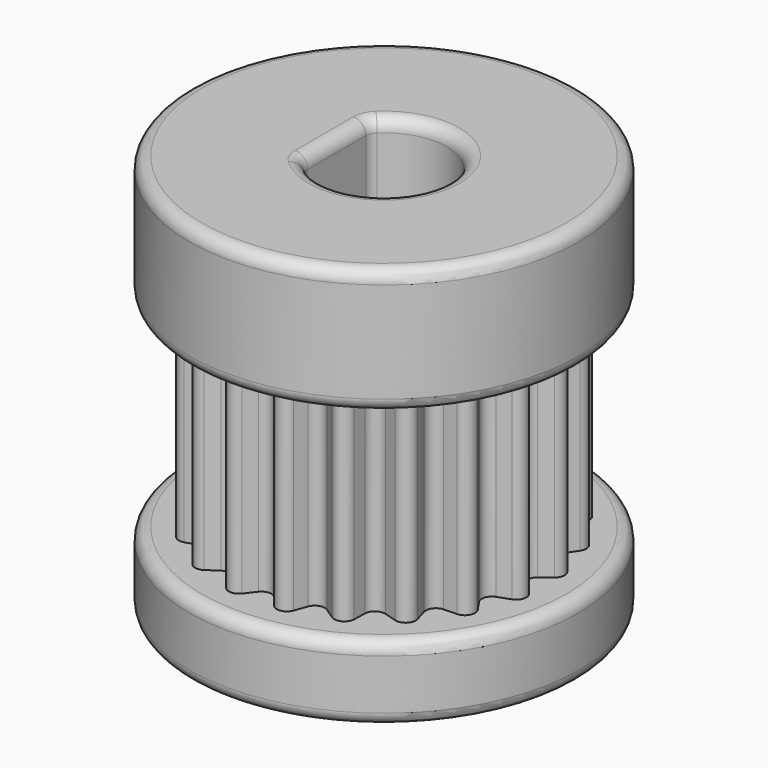
from build123d import *

# Parameters (mm, degrees)
F0_R     = 7.75
F1_DEPTH = 5
F2_DEPTH = 13
F3_START = -13
F3_DEPTH = 3
F4_R     = 0.5


with BuildPart() as f1:
    # F0 (on Top) → F1 (new body)
    with BuildSketch(Plane.XY):
        Circle(F0_R)
        with BuildLine():
            ThreePointArc((0.6382048465, 6.2700831172), (1.0168240228, 6.4199742139), (1.3305933613, 6.1604195498))
            Line((1.3305933613, 6.1604195498), (1.5086605411, 5.6659240772))
            ThreePointArc((1.5086605411, 5.6659240772), (1.7613968679, 5.4210221429), (2.1098145967, 5.4705972841))
            Line((2.1098145967, 5.4705972841), (2.5445311174, 5.7659872628))
            ThreePointArc((2.5445311174, 5.7659872628), (2.9509382483, 5.7915424072), (3.1691438202, 5.4477311947))
            Line((3.1691438202, 5.4477311947), (3.1856882672, 4.9224122685))
            ThreePointArc((3.1856882672, 4.9224122685), (3.3503759381, 4.6113968679), (3.6970604505, 4.5508786297))
            Line((3.6970604505, 4.5508786297), (4.2017809537, 4.6974764012))
            ThreePointArc((4.2017809537, 4.6974764012), (4.5961940777, 4.5961940777), (4.6974764012, 4.2017809537))
            Line((4.6974764012, 4.2017809537), (4.5508786297, 3.6970604505))
            ThreePointArc((4.5508786297, 3.6970604505), (4.6113968679, 3.3503759381), (4.9224122685, 3.1856882672))
            Line((4.9224122685, 3.1856882672), (5.4477311947, 3.1691438202))
            ThreePointArc((5.4477311947, 3.1691438202), (5.7915424072, 2.9509382483), (5.7659872628, 2.5445311174))
            Line((5.7659872628, 2.5445311174), (5.4705972841, 2.1098145967))
            ThreePointArc((5.4705972841, 2.1098145967), (5.4210221429, 1.7613968679), (5.6659240772, 1.5086605411))
            Line((5.6659240772, 1.5086605411), (6.1604195498, 1.3305933613))
            ThreePointArc((6.1604195498, 1.3305933613), (6.4199742139, 1.0168240228), (6.2700831172, 0.6382048465))
            Line((6.2700831172, 0.6382048465), (5.8548157604, 0.3160453902))
            ThreePointArc((5.8548157604, 0.3160453902), (5.7, 0), (5.8548157604, -0.3160453902))
            Line((5.8548157604, -0.3160453902), (6.2700831172, -0.6382048465))
            ThreePointArc((6.2700831172, -0.6382048465), (6.4199742139, -1.0168240228), (6.1604195498, -1.3305933613))
            Line((6.1604195498, -1.3305933613), (5.6659240772, -1.5086605411))
            ThreePointArc((5.6659240772, -1.5086605411), (5.4210221429, -1.7613968679), (5.4705972841, -2.1098145967))
            Line((5.4705972841, -2.1098145967), (5.7659872628, -2.5445311174))
            ThreePointArc((5.7659872628, -2.5445311174), (5.7915424072, -2.9509382483), (5.4477311947, -3.1691438202))
            Line((5.4477311947, -3.1691438202), (4.9224122685, -3.1856882672))
            ThreePointArc((4.9224122685, -3.1856882672), (4.6113968679, -3.3503759381), (4.5508786297, -3.6970604505))
            Line((4.5508786297, -3.6970604505), (4.6974764012, -4.2017809537))
            ThreePointArc((4.6974764012, -4.2017809537), (4.5961940777, -4.5961940777), (4.2017809537, -4.6974764012))
            Line((4.2017809537, -4.6974764012), (3.6970604505, -4.5508786297))
            ThreePointArc((3.6970604505, -4.5508786297), (3.3503759381, -4.6113968679), (3.1856882672, -4.9224122685))
            Line((3.1856882672, -4.9224122685), (3.1691438202, -5.4477311947))
            ThreePointArc((3.1691438202, -5.4477311947), (2.9509382483, -5.7915424072), (2.5445311174, -5.7659872628))
            Line((2.5445311174, -5.7659872628), (2.1098145967, -5.4705972841))
            ThreePointArc((2.1098145967, -5.4705972841), (1.7613968679, -5.4210221429), (1.5086605411, -5.6659240772))
            Line((1.5086605411, -5.6659240772), (1.3305933613, -6.1604195498))
            ThreePointArc((1.3305933613, -6.1604195498), (1.0168240228, -6.4199742139), (0.6382048465, -6.2700831172))
            Line((0.6382048465, -6.2700831172), (0.3160453902, -5.8548157604))
            ThreePointArc((0.3160453902, -5.8548157604), (0, -5.7), (-0.3160453902, -5.8548157604))
            Line((-0.3160453902, -5.8548157604), (-0.6382048465, -6.2700831172))
            ThreePointArc((-0.6382048465, -6.2700831172), (-1.0168240228, -6.4199742139), (-1.3305933613, -6.1604195498))
            Line((-1.3305933613, -6.1604195498), (-1.5086605411, -5.6659240772))
            ThreePointArc((-1.5086605411, -5.6659240772), (-1.7613968679, -5.4210221429), (-2.1098145967, -5.4705972841))
            Line((-2.1098145967, -5.4705972841), (-2.5445311174, -5.7659872628))
            ThreePointArc((-2.5445311174, -5.7659872628), (-2.9509382483, -5.7915424072), (-3.1691438202, -5.4477311947))
            Line((-3.1691438202, -5.4477311947), (-3.1856882672, -4.9224122685))
            ThreePointArc((-3.1856882672, -4.9224122685), (-3.3503759381, -4.6113968679), (-3.6970604505, -4.5508786297))
            Line((-3.6970604505, -4.5508786297), (-4.2017809537, -4.6974764012))
            ThreePointArc((-4.2017809537, -4.6974764012), (-4.5961940777, -4.5961940777), (-4.6974764012, -4.2017809537))
            Line((-4.6974764012, -4.2017809537), (-4.5508786297, -3.6970604505))
            ThreePointArc((-4.5508786297, -3.6970604505), (-4.6113968679, -3.3503759381), (-4.9224122685, -3.1856882672))
            Line((-4.9224122685, -3.1856882672), (-5.4477311947, -3.1691438202))
            ThreePointArc((-5.4477311947, -3.1691438202), (-5.7915424072, -2.9509382483), (-5.7659872628, -2.5445311174))
            Line((-5.7659872628, -2.5445311174), (-5.4705972841, -2.1098145967))
            ThreePointArc((-5.4705972841, -2.1098145967), (-5.4210221429, -1.7613968679), (-5.6659240772, -1.5086605411))
            Line((-5.6659240772, -1.5086605411), (-6.1604195498, -1.3305933613))
            ThreePointArc((-6.1604195498, -1.3305933613), (-6.4199742139, -1.0168240228), (-6.2700831172, -0.6382048465))
            Line((-6.2700831172, -0.6382048465), (-5.8548157604, -0.3160453902))
            ThreePointArc((-5.8548157604, -0.3160453902), (-5.7, 0), (-5.8548157604, 0.3160453902))
            Line((-5.8548157604, 0.3160453902), (-6.2700831172, 0.6382048465))
            ThreePointArc((-6.2700831172, 0.6382048465), (-6.4199742139, 1.0168240228), (-6.1604195498, 1.3305933613))
            Line((-6.1604195498, 1.3305933613), (-5.6659240772, 1.5086605411))
            ThreePointArc((-5.6659240772, 1.5086605411), (-5.4210221429, 1.7613968679), (-5.4705972841, 2.1098145967))
            Line((-5.4705972841, 2.1098145967), (-5.7659872628, 2.5445311174))
            ThreePointArc((-5.7659872628, 2.5445311174), (-5.7915424072, 2.9509382483), (-5.4477311947, 3.1691438202))
            Line((-5.4477311947, 3.1691438202), (-4.9224122685, 3.1856882672))
            ThreePointArc((-4.9224122685, 3.1856882672), (-4.6113968679, 3.3503759381), (-4.5508786297, 3.6970604505))
            Line((-4.5508786297, 3.6970604505), (-4.6974764012, 4.2017809537))
            ThreePointArc((-4.6974764012, 4.2017809537), (-4.5961940777, 4.5961940777), (-4.2017809537, 4.6974764012))
            Line((-4.2017809537, 4.6974764012), (-3.6970604505, 4.5508786297))
            ThreePointArc((-3.6970604505, 4.5508786297), (-3.3503759381, 4.6113968679), (-3.1856882672, 4.9224122685))
            Line((-3.1856882672, 4.9224122685), (-3.1691438202, 5.4477311947))
            ThreePointArc((-3.1691438202, 5.4477311947), (-2.9509382483, 5.7915424072), (-2.5445311174, 5.7659872628))
            Line((-2.5445311174, 5.7659872628), (-2.1098145967, 5.4705972841))
            ThreePointArc((-2.1098145967, 5.4705972841), (-1.7613968679, 5.4210221429), (-1.5086605411, 5.6659240772))
            Line((-1.5086605411, 5.6659240772), (-1.3305933613, 6.1604195498))
            ThreePointArc((-1.3305933613, 6.1604195498), (-1.0168240228, 6.4199742139), (-0.6382048465, 6.2700831172))
            Line((-0.6382048465, 6.2700831172), (-0.3160453902, 5.8548157604))
            ThreePointArc((-0.3160453902, 5.8548157604), (0, 5.7), (0.3160453902, 5.8548157604))
            Line((0.3160453902, 5.8548157604), (0.6382048465, 6.2700831172))
        make_face(mode=Mode.SUBTRACT)
        with BuildLine():
            Line((1.5086605411, 5.6659240772), (1.3305933613, 6.1604195498))
            ThreePointArc((1.3305933613, 6.1604195498), (1.0168240228, 6.4199742139), (0.6382048465, 6.2700831172))
            Line((0.6382048465, 6.2700831172), (0.3160453902, 5.8548157604))
            ThreePointArc((0.3160453902, 5.8548157604), (0, 5.7), (-0.3160453902, 5.8548157604))
            Line((-0.3160453902, 5.8548157604), (-0.6382048465, 6.2700831172))
            ThreePointArc((-0.6382048465, 6.2700831172), (-1.0168240228, 6.4199742139), (-1.3305933613, 6.1604195498))
            Line((-1.3305933613, 6.1604195498), (-1.5086605411, 5.6659240772))
            ThreePointArc((-1.5086605411, 5.6659240772), (-1.7613968679, 5.4210221429), (-2.1098145967, 5.4705972841))
            Line((-2.1098145967, 5.4705972841), (-2.5445311174, 5.7659872628))
            ThreePointArc((-2.5445311174, 5.7659872628), (-2.9509382483, 5.7915424072), (-3.1691438202, 5.4477311947))
            Line((-3.1691438202, 5.4477311947), (-3.1856882672, 4.9224122685))
            ThreePointArc((-3.1856882672, 4.9224122685), (-3.3503759381, 4.6113968679), (-3.6970604505, 4.5508786297))
            Line((-3.6970604505, 4.5508786297), (-4.2017809537, 4.6974764012))
            ThreePointArc((-4.2017809537, 4.6974764012), (-4.5961940777, 4.5961940777), (-4.6974764012, 4.2017809537))
            Line((-4.6974764012, 4.2017809537), (-4.5508786297, 3.6970604505))
            ThreePointArc((-4.5508786297, 3.6970604505), (-4.6113968679, 3.3503759381), (-4.9224122685, 3.1856882672))
            Line((-4.9224122685, 3.1856882672), (-5.4477311947, 3.1691438202))
            ThreePointArc((-5.4477311947, 3.1691438202), (-5.7915424072, 2.9509382483), (-5.7659872628, 2.5445311174))
            Line((-5.7659872628, 2.5445311174), (-5.4705972841, 2.1098145967))
            ThreePointArc((-5.4705972841, 2.1098145967), (-5.4210221429, 1.7613968679), (-5.6659240772, 1.5086605411))
            Line((-5.6659240772, 1.5086605411), (-6.1604195498, 1.3305933613))
            ThreePointArc((-6.1604195498, 1.3305933613), (-6.4199742139, 1.0168240228), (-6.2700831172, 0.6382048465))
            Line((-6.2700831172, 0.6382048465), (-5.8548157604, 0.3160453902))
            ThreePointArc((-5.8548157604, 0.3160453902), (-5.7, 0), (-5.8548157604, -0.3160453902))
            Line((-5.8548157604, -0.3160453902), (-6.2700831172, -0.6382048465))
            ThreePointArc((-6.2700831172, -0.6382048465), (-6.4199742139, -1.0168240228), (-6.1604195498, -1.3305933613))
            Line((-6.1604195498, -1.3305933613), (-5.6659240772, -1.5086605411))
            ThreePointArc((-5.6659240772, -1.5086605411), (-5.4210221429, -1.7613968679), (-5.4705972841, -2.1098145967))
            Line((-5.4705972841, -2.1098145967), (-5.7659872628, -2.5445311174))
            ThreePointArc((-5.7659872628, -2.5445311174), (-5.7915424072, -2.9509382483), (-5.4477311947, -3.1691438202))
            Line((-5.4477311947, -3.1691438202), (-4.9224122685, -3.1856882672))
            ThreePointArc((-4.9224122685, -3.1856882672), (-4.6113968679, -3.3503759381), (-4.5508786297, -3.6970604505))
            Line((-4.5508786297, -3.6970604505), (-4.6974764012, -4.2017809537))
            ThreePointArc((-4.6974764012, -4.2017809537), (-4.5961940777, -4.5961940777), (-4.2017809537, -4.6974764012))
            Line((-4.2017809537, -4.6974764012), (-3.6970604505, -4.5508786297))
            ThreePointArc((-3.6970604505, -4.5508786297), (-3.3503759381, -4.6113968679), (-3.1856882672, -4.9224122685))
            Line((-3.1856882672, -4.9224122685), (-3.1691438202, -5.4477311947))
            ThreePointArc((-3.1691438202, -5.4477311947), (-2.9509382483, -5.7915424072), (-2.5445311174, -5.7659872628))
            Line((-2.5445311174, -5.7659872628), (-2.1098145967, -5.4705972841))
            ThreePointArc((-2.1098145967, -5.4705972841), (-1.7613968679, -5.4210221429), (-1.5086605411, -5.6659240772))
            Line((-1.5086605411, -5.6659240772), (-1.3305933613, -6.1604195498))
            ThreePointArc((-1.3305933613, -6.1604195498), (-1.0168240228, -6.4199742139), (-0.6382048465, -6.2700831172))
            Line((-0.6382048465, -6.2700831172), (-0.3160453902, -5.8548157604))
            ThreePointArc((-0.3160453902, -5.8548157604), (0, -5.7), (0.3160453902, -5.8548157604))
            Line((0.3160453902, -5.8548157604), (0.6382048465, -6.2700831172))
            ThreePointArc((0.6382048465, -6.2700831172), (1.0168240228, -6.4199742139), (1.3305933613, -6.1604195498))
            Line((1.3305933613, -6.1604195498), (1.5086605411, -5.6659240772))
            ThreePointArc((1.5086605411, -5.6659240772), (1.7613968679, -5.4210221429), (2.1098145967, -5.4705972841))
            Line((2.1098145967, -5.4705972841), (2.5445311174, -5.7659872628))
            ThreePointArc((2.5445311174, -5.7659872628), (2.9509382483, -5.7915424072), (3.1691438202, -5.4477311947))
            Line((3.1691438202, -5.4477311947), (3.1856882672, -4.9224122685))
            ThreePointArc((3.1856882672, -4.9224122685), (3.3503759381, -4.6113968679), (3.6970604505, -4.5508786297))
            Line((3.6970604505, -4.5508786297), (4.2017809537, -4.6974764012))
            ThreePointArc((4.2017809537, -4.6974764012), (4.5961940777, -4.5961940777), (4.6974764012, -4.2017809537))
            Line((4.6974764012, -4.2017809537), (4.5508786297, -3.6970604505))
            ThreePointArc((4.5508786297, -3.6970604505), (4.6113968679, -3.3503759381), (4.9224122685, -3.1856882672))
            Line((4.9224122685, -3.1856882672), (5.4477311947, -3.1691438202))
            ThreePointArc((5.4477311947, -3.1691438202), (5.7915424072, -2.9509382483), (5.7659872628, -2.5445311174))
            Line((5.7659872628, -2.5445311174), (5.4705972841, -2.1098145967))
            ThreePointArc((5.4705972841, -2.1098145967), (5.4210221429, -1.7613968679), (5.6659240772, -1.5086605411))
            Line((5.6659240772, -1.5086605411), (6.1604195498, -1.3305933613))
            ThreePointArc((6.1604195498, -1.3305933613), (6.4199742139, -1.0168240228), (6.2700831172, -0.6382048465))
            Line((6.2700831172, -0.6382048465), (5.8548157604, -0.3160453902))
            ThreePointArc((5.8548157604, -0.3160453902), (5.7, 0), (5.8548157604, 0.3160453902))
            Line((5.8548157604, 0.3160453902), (6.2700831172, 0.6382048465))
            ThreePointArc((6.2700831172, 0.6382048465), (6.4199742139, 1.0168240228), (6.1604195498, 1.3305933613))
            Line((6.1604195498, 1.3305933613), (5.6659240772, 1.5086605411))
            ThreePointArc((5.6659240772, 1.5086605411), (5.4210221429, 1.7613968679), (5.4705972841, 2.1098145967))
            Line((5.4705972841, 2.1098145967), (5.7659872628, 2.5445311174))
            ThreePointArc((5.7659872628, 2.5445311174), (5.7915424072, 2.9509382483), (5.4477311947, 3.1691438202))
            Line((5.4477311947, 3.1691438202), (4.9224122685, 3.1856882672))
            ThreePointArc((4.9224122685, 3.1856882672), (4.6113968679, 3.3503759381), (4.5508786297, 3.6970604505))
            Line((4.5508786297, 3.6970604505), (4.6974764012, 4.2017809537))
            ThreePointArc((4.6974764012, 4.2017809537), (4.5961940777, 4.5961940777), (4.2017809537, 4.6974764012))
            Line((4.2017809537, 4.6974764012), (3.6970604505, 4.5508786297))
            ThreePointArc((3.6970604505, 4.5508786297), (3.3503759381, 4.6113968679), (3.1856882672, 4.9224122685))
            Line((3.1856882672, 4.9224122685), (3.1691438202, 5.4477311947))
            ThreePointArc((3.1691438202, 5.4477311947), (2.9509382483, 5.7915424072), (2.5445311174, 5.7659872628))
            Line((2.5445311174, 5.7659872628), (2.1098145967, 5.4705972841))
            ThreePointArc((2.1098145967, 5.4705972841), (1.7613968679, 5.4210221429), (1.5086605411, 5.6659240772))
        make_face()
        with BuildLine():
            ThreePointArc((-1.8781639971, 1.65), (2.5, 0), (-1.8781639971, -1.65))
            Line((-1.8781639971, -1.65), (-1.8781639971, 1.65))
        make_face(mode=Mode.SUBTRACT)
    extrude(amount=-F1_DEPTH)

    # F0 (on Top) → F2 (join)
    with BuildSketch(Plane.XY):
        with BuildLine():
            Line((1.5086605411, 5.6659240772), (1.3305933613, 6.1604195498))
            ThreePointArc((1.3305933613, 6.1604195498), (1.0168240228, 6.4199742139), (0.6382048465, 6.2700831172))
            Line((0.6382048465, 6.2700831172), (0.3160453902, 5.8548157604))
            ThreePointArc((0.3160453902, 5.8548157604), (0, 5.7), (-0.3160453902, 5.8548157604))
            Line((-0.3160453902, 5.8548157604), (-0.6382048465, 6.2700831172))
            ThreePointArc((-0.6382048465, 6.2700831172), (-1.0168240228, 6.4199742139), (-1.3305933613, 6.1604195498))
            Line((-1.3305933613, 6.1604195498), (-1.5086605411, 5.6659240772))
            ThreePointArc((-1.5086605411, 5.6659240772), (-1.7613968679, 5.4210221429), (-2.1098145967, 5.4705972841))
            Line((-2.1098145967, 5.4705972841), (-2.5445311174, 5.7659872628))
            ThreePointArc((-2.5445311174, 5.7659872628), (-2.9509382483, 5.7915424072), (-3.1691438202, 5.4477311947))
            Line((-3.1691438202, 5.4477311947), (-3.1856882672, 4.9224122685))
            ThreePointArc((-3.1856882672, 4.9224122685), (-3.3503759381, 4.6113968679), (-3.6970604505, 4.5508786297))
            Line((-3.6970604505, 4.5508786297), (-4.2017809537, 4.6974764012))
            ThreePointArc((-4.2017809537, 4.6974764012), (-4.5961940777, 4.5961940777), (-4.6974764012, 4.2017809537))
            Line((-4.6974764012, 4.2017809537), (-4.5508786297, 3.6970604505))
            ThreePointArc((-4.5508786297, 3.6970604505), (-4.6113968679, 3.3503759381), (-4.9224122685, 3.1856882672))
            Line((-4.9224122685, 3.1856882672), (-5.4477311947, 3.1691438202))
            ThreePointArc((-5.4477311947, 3.1691438202), (-5.7915424072, 2.9509382483), (-5.7659872628, 2.5445311174))
            Line((-5.7659872628, 2.5445311174), (-5.4705972841, 2.1098145967))
            ThreePointArc((-5.4705972841, 2.1098145967), (-5.4210221429, 1.7613968679), (-5.6659240772, 1.5086605411))
            Line((-5.6659240772, 1.5086605411), (-6.1604195498, 1.3305933613))
            ThreePointArc((-6.1604195498, 1.3305933613), (-6.4199742139, 1.0168240228), (-6.2700831172, 0.6382048465))
            Line((-6.2700831172, 0.6382048465), (-5.8548157604, 0.3160453902))
            ThreePointArc((-5.8548157604, 0.3160453902), (-5.7, 0), (-5.8548157604, -0.3160453902))
            Line((-5.8548157604, -0.3160453902), (-6.2700831172, -0.6382048465))
            ThreePointArc((-6.2700831172, -0.6382048465), (-6.4199742139, -1.0168240228), (-6.1604195498, -1.3305933613))
            Line((-6.1604195498, -1.3305933613), (-5.6659240772, -1.5086605411))
            ThreePointArc((-5.6659240772, -1.5086605411), (-5.4210221429, -1.7613968679), (-5.4705972841, -2.1098145967))
            Line((-5.4705972841, -2.1098145967), (-5.7659872628, -2.5445311174))
            ThreePointArc((-5.7659872628, -2.5445311174), (-5.7915424072, -2.9509382483), (-5.4477311947, -3.1691438202))
            Line((-5.4477311947, -3.1691438202), (-4.9224122685, -3.1856882672))
            ThreePointArc((-4.9224122685, -3.1856882672), (-4.6113968679, -3.3503759381), (-4.5508786297, -3.6970604505))
            Line((-4.5508786297, -3.6970604505), (-4.6974764012, -4.2017809537))
            ThreePointArc((-4.6974764012, -4.2017809537), (-4.5961940777, -4.5961940777), (-4.2017809537, -4.6974764012))
            Line((-4.2017809537, -4.6974764012), (-3.6970604505, -4.5508786297))
            ThreePointArc((-3.6970604505, -4.5508786297), (-3.3503759381, -4.6113968679), (-3.1856882672, -4.9224122685))
            Line((-3.1856882672, -4.9224122685), (-3.1691438202, -5.4477311947))
            ThreePointArc((-3.1691438202, -5.4477311947), (-2.9509382483, -5.7915424072), (-2.5445311174, -5.7659872628))
            Line((-2.5445311174, -5.7659872628), (-2.1098145967, -5.4705972841))
            ThreePointArc((-2.1098145967, -5.4705972841), (-1.7613968679, -5.4210221429), (-1.5086605411, -5.6659240772))
            Line((-1.5086605411, -5.6659240772), (-1.3305933613, -6.1604195498))
            ThreePointArc((-1.3305933613, -6.1604195498), (-1.0168240228, -6.4199742139), (-0.6382048465, -6.2700831172))
            Line((-0.6382048465, -6.2700831172), (-0.3160453902, -5.8548157604))
            ThreePointArc((-0.3160453902, -5.8548157604), (0, -5.7), (0.3160453902, -5.8548157604))
            Line((0.3160453902, -5.8548157604), (0.6382048465, -6.2700831172))
            ThreePointArc((0.6382048465, -6.2700831172), (1.0168240228, -6.4199742139), (1.3305933613, -6.1604195498))
            Line((1.3305933613, -6.1604195498), (1.5086605411, -5.6659240772))
            ThreePointArc((1.5086605411, -5.6659240772), (1.7613968679, -5.4210221429), (2.1098145967, -5.4705972841))
            Line((2.1098145967, -5.4705972841), (2.5445311174, -5.7659872628))
            ThreePointArc((2.5445311174, -5.7659872628), (2.9509382483, -5.7915424072), (3.1691438202, -5.4477311947))
            Line((3.1691438202, -5.4477311947), (3.1856882672, -4.9224122685))
            ThreePointArc((3.1856882672, -4.9224122685), (3.3503759381, -4.6113968679), (3.6970604505, -4.5508786297))
            Line((3.6970604505, -4.5508786297), (4.2017809537, -4.6974764012))
            ThreePointArc((4.2017809537, -4.6974764012), (4.5961940777, -4.5961940777), (4.6974764012, -4.2017809537))
            Line((4.6974764012, -4.2017809537), (4.5508786297, -3.6970604505))
            ThreePointArc((4.5508786297, -3.6970604505), (4.6113968679, -3.3503759381), (4.9224122685, -3.1856882672))
            Line((4.9224122685, -3.1856882672), (5.4477311947, -3.1691438202))
            ThreePointArc((5.4477311947, -3.1691438202), (5.7915424072, -2.9509382483), (5.7659872628, -2.5445311174))
            Line((5.7659872628, -2.5445311174), (5.4705972841, -2.1098145967))
            ThreePointArc((5.4705972841, -2.1098145967), (5.4210221429, -1.7613968679), (5.6659240772, -1.5086605411))
            Line((5.6659240772, -1.5086605411), (6.1604195498, -1.3305933613))
            ThreePointArc((6.1604195498, -1.3305933613), (6.4199742139, -1.0168240228), (6.2700831172, -0.6382048465))
            Line((6.2700831172, -0.6382048465), (5.8548157604, -0.3160453902))
            ThreePointArc((5.8548157604, -0.3160453902), (5.7, 0), (5.8548157604, 0.3160453902))
            Line((5.8548157604, 0.3160453902), (6.2700831172, 0.6382048465))
            ThreePointArc((6.2700831172, 0.6382048465), (6.4199742139, 1.0168240228), (6.1604195498, 1.3305933613))
            Line((6.1604195498, 1.3305933613), (5.6659240772, 1.5086605411))
            ThreePointArc((5.6659240772, 1.5086605411), (5.4210221429, 1.7613968679), (5.4705972841, 2.1098145967))
            Line((5.4705972841, 2.1098145967), (5.7659872628, 2.5445311174))
            ThreePointArc((5.7659872628, 2.5445311174), (5.7915424072, 2.9509382483), (5.4477311947, 3.1691438202))
            Line((5.4477311947, 3.1691438202), (4.9224122685, 3.1856882672))
            ThreePointArc((4.9224122685, 3.1856882672), (4.6113968679, 3.3503759381), (4.5508786297, 3.6970604505))
            Line((4.5508786297, 3.6970604505), (4.6974764012, 4.2017809537))
            ThreePointArc((4.6974764012, 4.2017809537), (4.5961940777, 4.5961940777), (4.2017809537, 4.6974764012))
            Line((4.2017809537, 4.6974764012), (3.6970604505, 4.5508786297))
            ThreePointArc((3.6970604505, 4.5508786297), (3.3503759381, 4.6113968679), (3.1856882672, 4.9224122685))
            Line((3.1856882672, 4.9224122685), (3.1691438202, 5.4477311947))
            ThreePointArc((3.1691438202, 5.4477311947), (2.9509382483, 5.7915424072), (2.5445311174, 5.7659872628))
            Line((2.5445311174, 5.7659872628), (2.1098145967, 5.4705972841))
            ThreePointArc((2.1098145967, 5.4705972841), (1.7613968679, 5.4210221429), (1.5086605411, 5.6659240772))
        make_face()
        with BuildLine():
            ThreePointArc((-1.8781639971, 1.65), (2.5, 0), (-1.8781639971, -1.65))
            Line((-1.8781639971, -1.65), (-1.8781639971, 1.65))
        make_face(mode=Mode.SUBTRACT)
    extrude(amount=-F2_DEPTH)

    # F0 (on Top) → F3 (join)
    with BuildSketch(Plane.XY.offset(F3_START)):
        Circle(F0_R)
        with BuildLine():
            ThreePointArc((0.6382048465, 6.2700831172), (1.0168240228, 6.4199742139), (1.3305933613, 6.1604195498))
            Line((1.3305933613, 6.1604195498), (1.5086605411, 5.6659240772))
            ThreePointArc((1.5086605411, 5.6659240772), (1.7613968679, 5.4210221429), (2.1098145967, 5.4705972841))
            Line((2.1098145967, 5.4705972841), (2.5445311174, 5.7659872628))
            ThreePointArc((2.5445311174, 5.7659872628), (2.9509382483, 5.7915424072), (3.1691438202, 5.4477311947))
            Line((3.1691438202, 5.4477311947), (3.1856882672, 4.9224122685))
            ThreePointArc((3.1856882672, 4.9224122685), (3.3503759381, 4.6113968679), (3.6970604505, 4.5508786297))
            Line((3.6970604505, 4.5508786297), (4.2017809537, 4.6974764012))
            ThreePointArc((4.2017809537, 4.6974764012), (4.5961940777, 4.5961940777), (4.6974764012, 4.2017809537))
            Line((4.6974764012, 4.2017809537), (4.5508786297, 3.6970604505))
            ThreePointArc((4.5508786297, 3.6970604505), (4.6113968679, 3.3503759381), (4.9224122685, 3.1856882672))
            Line((4.9224122685, 3.1856882672), (5.4477311947, 3.1691438202))
            ThreePointArc((5.4477311947, 3.1691438202), (5.7915424072, 2.9509382483), (5.7659872628, 2.5445311174))
            Line((5.7659872628, 2.5445311174), (5.4705972841, 2.1098145967))
            ThreePointArc((5.4705972841, 2.1098145967), (5.4210221429, 1.7613968679), (5.6659240772, 1.5086605411))
            Line((5.6659240772, 1.5086605411), (6.1604195498, 1.3305933613))
            ThreePointArc((6.1604195498, 1.3305933613), (6.4199742139, 1.0168240228), (6.2700831172, 0.6382048465))
            Line((6.2700831172, 0.6382048465), (5.8548157604, 0.3160453902))
            ThreePointArc((5.8548157604, 0.3160453902), (5.7, 0), (5.8548157604, -0.3160453902))
            Line((5.8548157604, -0.3160453902), (6.2700831172, -0.6382048465))
            ThreePointArc((6.2700831172, -0.6382048465), (6.4199742139, -1.0168240228), (6.1604195498, -1.3305933613))
            Line((6.1604195498, -1.3305933613), (5.6659240772, -1.5086605411))
            ThreePointArc((5.6659240772, -1.5086605411), (5.4210221429, -1.7613968679), (5.4705972841, -2.1098145967))
            Line((5.4705972841, -2.1098145967), (5.7659872628, -2.5445311174))
            ThreePointArc((5.7659872628, -2.5445311174), (5.7915424072, -2.9509382483), (5.4477311947, -3.1691438202))
            Line((5.4477311947, -3.1691438202), (4.9224122685, -3.1856882672))
            ThreePointArc((4.9224122685, -3.1856882672), (4.6113968679, -3.3503759381), (4.5508786297, -3.6970604505))
            Line((4.5508786297, -3.6970604505), (4.6974764012, -4.2017809537))
            ThreePointArc((4.6974764012, -4.2017809537), (4.5961940777, -4.5961940777), (4.2017809537, -4.6974764012))
            Line((4.2017809537, -4.6974764012), (3.6970604505, -4.5508786297))
            ThreePointArc((3.6970604505, -4.5508786297), (3.3503759381, -4.6113968679), (3.1856882672, -4.9224122685))
            Line((3.1856882672, -4.9224122685), (3.1691438202, -5.4477311947))
            ThreePointArc((3.1691438202, -5.4477311947), (2.9509382483, -5.7915424072), (2.5445311174, -5.7659872628))
            Line((2.5445311174, -5.7659872628), (2.1098145967, -5.4705972841))
            ThreePointArc((2.1098145967, -5.4705972841), (1.7613968679, -5.4210221429), (1.5086605411, -5.6659240772))
            Line((1.5086605411, -5.6659240772), (1.3305933613, -6.1604195498))
            ThreePointArc((1.3305933613, -6.1604195498), (1.0168240228, -6.4199742139), (0.6382048465, -6.2700831172))
            Line((0.6382048465, -6.2700831172), (0.3160453902, -5.8548157604))
            ThreePointArc((0.3160453902, -5.8548157604), (0, -5.7), (-0.3160453902, -5.8548157604))
            Line((-0.3160453902, -5.8548157604), (-0.6382048465, -6.2700831172))
            ThreePointArc((-0.6382048465, -6.2700831172), (-1.0168240228, -6.4199742139), (-1.3305933613, -6.1604195498))
            Line((-1.3305933613, -6.1604195498), (-1.5086605411, -5.6659240772))
            ThreePointArc((-1.5086605411, -5.6659240772), (-1.7613968679, -5.4210221429), (-2.1098145967, -5.4705972841))
            Line((-2.1098145967, -5.4705972841), (-2.5445311174, -5.7659872628))
            ThreePointArc((-2.5445311174, -5.7659872628), (-2.9509382483, -5.7915424072), (-3.1691438202, -5.4477311947))
            Line((-3.1691438202, -5.4477311947), (-3.1856882672, -4.9224122685))
            ThreePointArc((-3.1856882672, -4.9224122685), (-3.3503759381, -4.6113968679), (-3.6970604505, -4.5508786297))
            Line((-3.6970604505, -4.5508786297), (-4.2017809537, -4.6974764012))
            ThreePointArc((-4.2017809537, -4.6974764012), (-4.5961940777, -4.5961940777), (-4.6974764012, -4.2017809537))
            Line((-4.6974764012, -4.2017809537), (-4.5508786297, -3.6970604505))
            ThreePointArc((-4.5508786297, -3.6970604505), (-4.6113968679, -3.3503759381), (-4.9224122685, -3.1856882672))
            Line((-4.9224122685, -3.1856882672), (-5.4477311947, -3.1691438202))
            ThreePointArc((-5.4477311947, -3.1691438202), (-5.7915424072, -2.9509382483), (-5.7659872628, -2.5445311174))
            Line((-5.7659872628, -2.5445311174), (-5.4705972841, -2.1098145967))
            ThreePointArc((-5.4705972841, -2.1098145967), (-5.4210221429, -1.7613968679), (-5.6659240772, -1.5086605411))
            Line((-5.6659240772, -1.5086605411), (-6.1604195498, -1.3305933613))
            ThreePointArc((-6.1604195498, -1.3305933613), (-6.4199742139, -1.0168240228), (-6.2700831172, -0.6382048465))
            Line((-6.2700831172, -0.6382048465), (-5.8548157604, -0.3160453902))
            ThreePointArc((-5.8548157604, -0.3160453902), (-5.7, 0), (-5.8548157604, 0.3160453902))
            Line((-5.8548157604, 0.3160453902), (-6.2700831172, 0.6382048465))
            ThreePointArc((-6.2700831172, 0.6382048465), (-6.4199742139, 1.0168240228), (-6.1604195498, 1.3305933613))
            Line((-6.1604195498, 1.3305933613), (-5.6659240772, 1.5086605411))
            ThreePointArc((-5.6659240772, 1.5086605411), (-5.4210221429, 1.7613968679), (-5.4705972841, 2.1098145967))
            Line((-5.4705972841, 2.1098145967), (-5.7659872628, 2.5445311174))
            ThreePointArc((-5.7659872628, 2.5445311174), (-5.7915424072, 2.9509382483), (-5.4477311947, 3.1691438202))
            Line((-5.4477311947, 3.1691438202), (-4.9224122685, 3.1856882672))
            ThreePointArc((-4.9224122685, 3.1856882672), (-4.6113968679, 3.3503759381), (-4.5508786297, 3.6970604505))
            Line((-4.5508786297, 3.6970604505), (-4.6974764012, 4.2017809537))
            ThreePointArc((-4.6974764012, 4.2017809537), (-4.5961940777, 4.5961940777), (-4.2017809537, 4.6974764012))
            Line((-4.2017809537, 4.6974764012), (-3.6970604505, 4.5508786297))
            ThreePointArc((-3.6970604505, 4.5508786297), (-3.3503759381, 4.6113968679), (-3.1856882672, 4.9224122685))
            Line((-3.1856882672, 4.9224122685), (-3.1691438202, 5.4477311947))
            ThreePointArc((-3.1691438202, 5.4477311947), (-2.9509382483, 5.7915424072), (-2.5445311174, 5.7659872628))
            Line((-2.5445311174, 5.7659872628), (-2.1098145967, 5.4705972841))
            ThreePointArc((-2.1098145967, 5.4705972841), (-1.7613968679, 5.4210221429), (-1.5086605411, 5.6659240772))
            Line((-1.5086605411, 5.6659240772), (-1.3305933613, 6.1604195498))
            ThreePointArc((-1.3305933613, 6.1604195498), (-1.0168240228, 6.4199742139), (-0.6382048465, 6.2700831172))
            Line((-0.6382048465, 6.2700831172), (-0.3160453902, 5.8548157604))
            ThreePointArc((-0.3160453902, 5.8548157604), (0, 5.7), (0.3160453902, 5.8548157604))
            Line((0.3160453902, 5.8548157604), (0.6382048465, 6.2700831172))
        make_face(mode=Mode.SUBTRACT)
        with BuildLine():
            Line((1.5086605411, 5.6659240772), (1.3305933613, 6.1604195498))
            ThreePointArc((1.3305933613, 6.1604195498), (1.0168240228, 6.4199742139), (0.6382048465, 6.2700831172))
            Line((0.6382048465, 6.2700831172), (0.3160453902, 5.8548157604))
            ThreePointArc((0.3160453902, 5.8548157604), (0, 5.7), (-0.3160453902, 5.8548157604))
            Line((-0.3160453902, 5.8548157604), (-0.6382048465, 6.2700831172))
            ThreePointArc((-0.6382048465, 6.2700831172), (-1.0168240228, 6.4199742139), (-1.3305933613, 6.1604195498))
            Line((-1.3305933613, 6.1604195498), (-1.5086605411, 5.6659240772))
            ThreePointArc((-1.5086605411, 5.6659240772), (-1.7613968679, 5.4210221429), (-2.1098145967, 5.4705972841))
            Line((-2.1098145967, 5.4705972841), (-2.5445311174, 5.7659872628))
            ThreePointArc((-2.5445311174, 5.7659872628), (-2.9509382483, 5.7915424072), (-3.1691438202, 5.4477311947))
            Line((-3.1691438202, 5.4477311947), (-3.1856882672, 4.9224122685))
            ThreePointArc((-3.1856882672, 4.9224122685), (-3.3503759381, 4.6113968679), (-3.6970604505, 4.5508786297))
            Line((-3.6970604505, 4.5508786297), (-4.2017809537, 4.6974764012))
            ThreePointArc((-4.2017809537, 4.6974764012), (-4.5961940777, 4.5961940777), (-4.6974764012, 4.2017809537))
            Line((-4.6974764012, 4.2017809537), (-4.5508786297, 3.6970604505))
            ThreePointArc((-4.5508786297, 3.6970604505), (-4.6113968679, 3.3503759381), (-4.9224122685, 3.1856882672))
            Line((-4.9224122685, 3.1856882672), (-5.4477311947, 3.1691438202))
            ThreePointArc((-5.4477311947, 3.1691438202), (-5.7915424072, 2.9509382483), (-5.7659872628, 2.5445311174))
            Line((-5.7659872628, 2.5445311174), (-5.4705972841, 2.1098145967))
            ThreePointArc((-5.4705972841, 2.1098145967), (-5.4210221429, 1.7613968679), (-5.6659240772, 1.5086605411))
            Line((-5.6659240772, 1.5086605411), (-6.1604195498, 1.3305933613))
            ThreePointArc((-6.1604195498, 1.3305933613), (-6.4199742139, 1.0168240228), (-6.2700831172, 0.6382048465))
            Line((-6.2700831172, 0.6382048465), (-5.8548157604, 0.3160453902))
            ThreePointArc((-5.8548157604, 0.3160453902), (-5.7, 0), (-5.8548157604, -0.3160453902))
            Line((-5.8548157604, -0.3160453902), (-6.2700831172, -0.6382048465))
            ThreePointArc((-6.2700831172, -0.6382048465), (-6.4199742139, -1.0168240228), (-6.1604195498, -1.3305933613))
            Line((-6.1604195498, -1.3305933613), (-5.6659240772, -1.5086605411))
            ThreePointArc((-5.6659240772, -1.5086605411), (-5.4210221429, -1.7613968679), (-5.4705972841, -2.1098145967))
            Line((-5.4705972841, -2.1098145967), (-5.7659872628, -2.5445311174))
            ThreePointArc((-5.7659872628, -2.5445311174), (-5.7915424072, -2.9509382483), (-5.4477311947, -3.1691438202))
            Line((-5.4477311947, -3.1691438202), (-4.9224122685, -3.1856882672))
            ThreePointArc((-4.9224122685, -3.1856882672), (-4.6113968679, -3.3503759381), (-4.5508786297, -3.6970604505))
            Line((-4.5508786297, -3.6970604505), (-4.6974764012, -4.2017809537))
            ThreePointArc((-4.6974764012, -4.2017809537), (-4.5961940777, -4.5961940777), (-4.2017809537, -4.6974764012))
            Line((-4.2017809537, -4.6974764012), (-3.6970604505, -4.5508786297))
            ThreePointArc((-3.6970604505, -4.5508786297), (-3.3503759381, -4.6113968679), (-3.1856882672, -4.9224122685))
            Line((-3.1856882672, -4.9224122685), (-3.1691438202, -5.4477311947))
            ThreePointArc((-3.1691438202, -5.4477311947), (-2.9509382483, -5.7915424072), (-2.5445311174, -5.7659872628))
            Line((-2.5445311174, -5.7659872628), (-2.1098145967, -5.4705972841))
            ThreePointArc((-2.1098145967, -5.4705972841), (-1.7613968679, -5.4210221429), (-1.5086605411, -5.6659240772))
            Line((-1.5086605411, -5.6659240772), (-1.3305933613, -6.1604195498))
            ThreePointArc((-1.3305933613, -6.1604195498), (-1.0168240228, -6.4199742139), (-0.6382048465, -6.2700831172))
            Line((-0.6382048465, -6.2700831172), (-0.3160453902, -5.8548157604))
            ThreePointArc((-0.3160453902, -5.8548157604), (0, -5.7), (0.3160453902, -5.8548157604))
            Line((0.3160453902, -5.8548157604), (0.6382048465, -6.2700831172))
            ThreePointArc((0.6382048465, -6.2700831172), (1.0168240228, -6.4199742139), (1.3305933613, -6.1604195498))
            Line((1.3305933613, -6.1604195498), (1.5086605411, -5.6659240772))
            ThreePointArc((1.5086605411, -5.6659240772), (1.7613968679, -5.4210221429), (2.1098145967, -5.4705972841))
            Line((2.1098145967, -5.4705972841), (2.5445311174, -5.7659872628))
            ThreePointArc((2.5445311174, -5.7659872628), (2.9509382483, -5.7915424072), (3.1691438202, -5.4477311947))
            Line((3.1691438202, -5.4477311947), (3.1856882672, -4.9224122685))
            ThreePointArc((3.1856882672, -4.9224122685), (3.3503759381, -4.6113968679), (3.6970604505, -4.5508786297))
            Line((3.6970604505, -4.5508786297), (4.2017809537, -4.6974764012))
            ThreePointArc((4.2017809537, -4.6974764012), (4.5961940777, -4.5961940777), (4.6974764012, -4.2017809537))
            Line((4.6974764012, -4.2017809537), (4.5508786297, -3.6970604505))
            ThreePointArc((4.5508786297, -3.6970604505), (4.6113968679, -3.3503759381), (4.9224122685, -3.1856882672))
            Line((4.9224122685, -3.1856882672), (5.4477311947, -3.1691438202))
            ThreePointArc((5.4477311947, -3.1691438202), (5.7915424072, -2.9509382483), (5.7659872628, -2.5445311174))
            Line((5.7659872628, -2.5445311174), (5.4705972841, -2.1098145967))
            ThreePointArc((5.4705972841, -2.1098145967), (5.4210221429, -1.7613968679), (5.6659240772, -1.5086605411))
            Line((5.6659240772, -1.5086605411), (6.1604195498, -1.3305933613))
            ThreePointArc((6.1604195498, -1.3305933613), (6.4199742139, -1.0168240228), (6.2700831172, -0.6382048465))
            Line((6.2700831172, -0.6382048465), (5.8548157604, -0.3160453902))
            ThreePointArc((5.8548157604, -0.3160453902), (5.7, 0), (5.8548157604, 0.3160453902))
            Line((5.8548157604, 0.3160453902), (6.2700831172, 0.6382048465))
            ThreePointArc((6.2700831172, 0.6382048465), (6.4199742139, 1.0168240228), (6.1604195498, 1.3305933613))
            Line((6.1604195498, 1.3305933613), (5.6659240772, 1.5086605411))
            ThreePointArc((5.6659240772, 1.5086605411), (5.4210221429, 1.7613968679), (5.4705972841, 2.1098145967))
            Line((5.4705972841, 2.1098145967), (5.7659872628, 2.5445311174))
            ThreePointArc((5.7659872628, 2.5445311174), (5.7915424072, 2.9509382483), (5.4477311947, 3.1691438202))
            Line((5.4477311947, 3.1691438202), (4.9224122685, 3.1856882672))
            ThreePointArc((4.9224122685, 3.1856882672), (4.6113968679, 3.3503759381), (4.5508786297, 3.6970604505))
            Line((4.5508786297, 3.6970604505), (4.6974764012, 4.2017809537))
            ThreePointArc((4.6974764012, 4.2017809537), (4.5961940777, 4.5961940777), (4.2017809537, 4.6974764012))
            Line((4.2017809537, 4.6974764012), (3.6970604505, 4.5508786297))
            ThreePointArc((3.6970604505, 4.5508786297), (3.3503759381, 4.6113968679), (3.1856882672, 4.9224122685))
            Line((3.1856882672, 4.9224122685), (3.1691438202, 5.4477311947))
            ThreePointArc((3.1691438202, 5.4477311947), (2.9509382483, 5.7915424072), (2.5445311174, 5.7659872628))
            Line((2.5445311174, 5.7659872628), (2.1098145967, 5.4705972841))
            ThreePointArc((2.1098145967, 5.4705972841), (1.7613968679, 5.4210221429), (1.5086605411, 5.6659240772))
        make_face()
        with BuildLine():
            ThreePointArc((-1.8781639971, 1.65), (2.5, 0), (-1.8781639971, -1.65))
            Line((-1.8781639971, -1.65), (-1.8781639971, 1.65))
        make_face(mode=Mode.SUBTRACT)
    extrude(amount=-F3_DEPTH)

    # F4
    f4_edges = [f1.edges().sort_by_distance(p)[0] for p in [
        (-7.75, 0, 0),
        (-7.75, 0, -5),
        (-7.75, 0, -13),
        (-7.75, 0, -16),
        (2.5, 0, 0),
        (-1.878164, 0, 0),
        (-1.878164, 1.65, -8),
        (-1.878164, -1.65, -8),
        (2.5, 0, -16),
        (-1.878164, 0, -16),
    ]]
    fillet(f4_edges, radius=F4_R)


solid = f1.part
